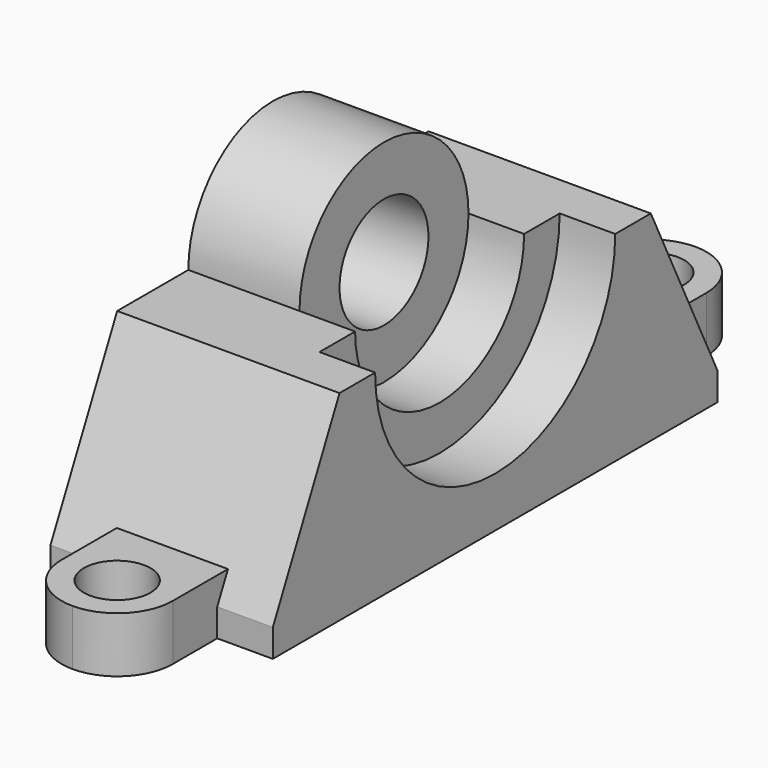
from build123d import *

# Parameters (mm, degrees)
F0_W         = 100
F0_H         = 36
F1_DEPTH     = 20
F2_W         = 20
F2_H         = 20
F3_DEPTH     = 10
F4_R         = 9.99999
F5_T4_DEPTH  = 200.6036926139
F5_T10_DEPTH = 200.6036926139
F5_T16_DEPTH = 200.6036926139
F5_T23_DEPTH = 200.6036926139
F5_T29_DEPTH = 200.6036926139
F6_R         = 6
F7_DEPTH     = 10.001
F8_T4_DEPTH  = 200.6036926139
F8_T10_DEPTH = 200.6036926139
F8_T16_DEPTH = 200.6036926139
F8_T23_DEPTH = 200.6036926139
F8_T29_DEPTH = 200.6036926139
F9_R         = 27
F10_DEPTH    = 10
F11_R        = 19
F12_DEPTH    = 10
F13_R        = 19
F14_DEPTH    = 20
F15_R        = 10
F16_DEPTH    = 20.001


# Not quite as in the source:
# - a fillet or chamfer that OpenCascade refuses, or shapes differently, is made with other operations: its cross-section is extruded or revolved along the edge and cut away or added
# - a fillet or chamfer is up to 0.001 mm smaller than in the source, because OpenCascade refuses the exact size
# - a pattern or mirror of a feature is missing from the dataset's text; its kind, count and spacing are read off the source's solid


with BuildPart() as f1:
    # F0 (on Right) → F1 (new body, symmetric)
    with BuildSketch(Plane.YZ):
        Rectangle(F0_W, F0_H)
    extrude(amount=F1_DEPTH, both=True)

    # F2 (on face) → F3 (join)
    with BuildSketch(Plane(origin=(0, 0, -18), x_dir=(1, 0, 0), z_dir=(0, 0, -1))):
        with Locations((0, 60)):
            Rectangle(F2_W, F2_H)
    f3 = extrude(amount=-F3_DEPTH)

    # F3_copies: F3 across plane
    add(f3.mirror(Plane.ZX.offset(-3e-06)))

    # F4 (radius 10 in the source; OpenCascade refuses exactly that, so slightly less here)
    f4_edges = [f1.edges().sort_by_distance(p)[0] for p in [
        (10, -70, -13),
        (-10, -70, -13),
        (-10, 69.999994, -13),
        (10, 69.999994, -13),
    ]]
    fillet(f4_edges, radius=F4_R)

    # F5: chamfer of 15 x 31 on 1 edges, made by hand


with BuildPart() as f5_tool2:
    # F5_s3 → F5_t4 (new body)
    with BuildSketch(Plane.YZ.offset(-100.301846307)):
        Polygon((-50, -13), (-35, 18), (-50, 18), align=None)
    extrude(amount=F5_T4_DEPTH)

    split(bisect_by=Plane.XY.offset(-8), keep=Keep.BOTTOM)

    split(bisect_by=Plane.YZ.offset(-10), keep=Keep.BOTTOM)


with BuildPart() as f1_1:
    add(f1.part)

    # F5_t1: cut F5_tool2
    add(f5_tool2.part, mode=Mode.SUBTRACT)


with BuildPart() as f5_tool8:
    # F5_s9 → F5_t10 (new body)
    with BuildSketch(Plane.YZ.offset(-100.301846307)):
        Polygon((-50, -13), (-35, 18), (-50, 18), align=None)
    extrude(amount=F5_T10_DEPTH)

    split(bisect_by=Plane.XY.offset(-8), keep=Keep.TOP)

    split(bisect_by=Plane.YZ.offset(-10), keep=Keep.BOTTOM)


with BuildPart() as f1_2:
    add(f1_1.part)

    # F5_t7: cut F5_tool8
    add(f5_tool8.part, mode=Mode.SUBTRACT)


with BuildPart() as f5_tool14:
    # F5_s15 → F5_t16 (new body)
    with BuildSketch(Plane.YZ.offset(-100.301846307)):
        Polygon((-50, -13), (-35, 18), (-50, 18), align=None)
    extrude(amount=F5_T16_DEPTH)

    split(bisect_by=Plane.YZ.offset(10), keep=Keep.BOTTOM)

    split(bisect_by=Plane.XY.offset(-8), keep=Keep.TOP)

    split(bisect_by=Plane.YZ.offset(-10), keep=Keep.TOP)


with BuildPart() as f1_3:
    add(f1_2.part)

    # F5_t13: cut F5_tool14
    add(f5_tool14.part, mode=Mode.SUBTRACT)


with BuildPart() as f5_tool21:
    # F5_s22 → F5_t23 (new body)
    with BuildSketch(Plane.YZ.offset(-100.301846307)):
        Polygon((-50, -13), (-35, 18), (-50, 18), align=None)
    extrude(amount=F5_T23_DEPTH)

    split(bisect_by=Plane.YZ.offset(10), keep=Keep.TOP)

    split(bisect_by=Plane.XY.offset(-8), keep=Keep.BOTTOM)


with BuildPart() as f1_4:
    add(f1_3.part)

    # F5_t20: cut F5_tool21
    add(f5_tool21.part, mode=Mode.SUBTRACT)


with BuildPart() as f5_tool27:
    # F5_s28 → F5_t29 (new body)
    with BuildSketch(Plane.YZ.offset(-100.301846307)):
        Polygon((-50, -13), (-35, 18), (-50, 18), align=None)
    extrude(amount=F5_T29_DEPTH)

    split(bisect_by=Plane.YZ.offset(10), keep=Keep.TOP)

    split(bisect_by=Plane.XY.offset(-8), keep=Keep.TOP)


with BuildPart() as f1_5:
    add(f1_4.part)

    # F5_t26: cut F5_tool27
    add(f5_tool27.part, mode=Mode.SUBTRACT)

    # F6 (on face) → F7 (cut, through all)
    with BuildSketch(Plane.XY.offset(-8)):
        with Locations((0, -60)):
            Circle(F6_R)
    f7 = extrude(amount=-F7_DEPTH, mode=Mode.SUBTRACT)

    # F7_copies: F7 across plane
    add(f7.mirror(Plane.ZX), mode=Mode.SUBTRACT)

    # F8: chamfer of 15 x 31 on 1 edges, made by hand


with BuildPart() as f8_tool2:
    # F8_s3 → F8_t4 (new body)
    with BuildSketch(Plane.YZ.offset(100.301846307)):
        Polygon((50, -13), (35, 18), (50, 18), align=None)
    extrude(amount=-F8_T4_DEPTH)

    split(bisect_by=Plane.XY.offset(-8), keep=Keep.BOTTOM)

    split(bisect_by=Plane.YZ.offset(10), keep=Keep.TOP)


with BuildPart() as f1_6:
    add(f1_5.part)

    # F8_t1: cut F8_tool2
    add(f8_tool2.part, mode=Mode.SUBTRACT)


with BuildPart() as f8_tool8:
    # F8_s9 → F8_t10 (new body)
    with BuildSketch(Plane.YZ.offset(100.301846307)):
        Polygon((50, -13), (35, 18), (50, 18), align=None)
    extrude(amount=-F8_T10_DEPTH)

    split(bisect_by=Plane.XY.offset(-8), keep=Keep.TOP)

    split(bisect_by=Plane.YZ.offset(10), keep=Keep.TOP)


with BuildPart() as f1_7:
    add(f1_6.part)

    # F8_t7: cut F8_tool8
    add(f8_tool8.part, mode=Mode.SUBTRACT)


with BuildPart() as f8_tool14:
    # F8_s15 → F8_t16 (new body)
    with BuildSketch(Plane.YZ.offset(100.301846307)):
        Polygon((50, -13), (35, 18), (50, 18), align=None)
    extrude(amount=-F8_T16_DEPTH)

    split(bisect_by=Plane.YZ.offset(-10), keep=Keep.TOP)

    split(bisect_by=Plane.XY.offset(-8), keep=Keep.TOP)

    split(bisect_by=Plane.YZ.offset(10), keep=Keep.BOTTOM)


with BuildPart() as f1_8:
    add(f1_7.part)

    # F8_t13: cut F8_tool14
    add(f8_tool14.part, mode=Mode.SUBTRACT)


with BuildPart() as f8_tool21:
    # F8_s22 → F8_t23 (new body)
    with BuildSketch(Plane.YZ.offset(100.301846307)):
        Polygon((50, -13), (35, 18), (50, 18), align=None)
    extrude(amount=-F8_T23_DEPTH)

    split(bisect_by=Plane.YZ.offset(-10), keep=Keep.BOTTOM)

    split(bisect_by=Plane.XY.offset(-8), keep=Keep.BOTTOM)


with BuildPart() as f1_9:
    add(f1_8.part)

    # F8_t20: cut F8_tool21
    add(f8_tool21.part, mode=Mode.SUBTRACT)


with BuildPart() as f8_tool27:
    # F8_s28 → F8_t29 (new body)
    with BuildSketch(Plane.YZ.offset(100.301846307)):
        Polygon((50, -13), (35, 18), (50, 18), align=None)
    extrude(amount=-F8_T29_DEPTH)

    split(bisect_by=Plane.YZ.offset(-10), keep=Keep.BOTTOM)

    split(bisect_by=Plane.XY.offset(-8), keep=Keep.TOP)


with BuildPart() as f1_10:
    add(f1_9.part)

    # F8_t26: cut F8_tool27
    add(f8_tool27.part, mode=Mode.SUBTRACT)

    # F9 (on face) → F10 (cut)
    with BuildSketch(Plane.YZ.offset(20)):
        with Locations((0, 18)):
            Circle(F9_R)
    extrude(amount=-F10_DEPTH, mode=Mode.SUBTRACT)

    # F11 (on face) → F12 (cut)
    with BuildSketch(Plane.YZ.offset(10)):
        with Locations((0, 18)):
            Circle(F11_R)
    extrude(amount=-F12_DEPTH, mode=Mode.SUBTRACT)

    # F13 (on face) → F14 (join)
    with BuildSketch(Plane.YZ):
        with Locations((0, 18)):
            Circle(F13_R)
    extrude(amount=-F14_DEPTH)

    # F15 (on face) → F16 (cut, through all)
    with BuildSketch(Plane.YZ):
        with Locations((0, 18)):
            Circle(F15_R)
    extrude(amount=-F16_DEPTH, mode=Mode.SUBTRACT)


solid = f1_10.part
